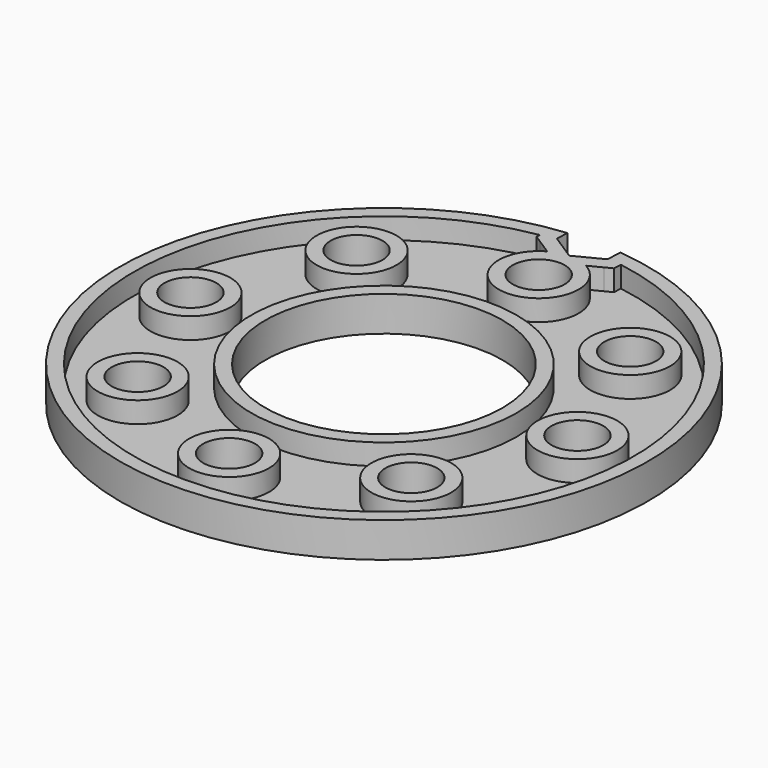
from build123d import *

# Parameters (mm, degrees)
F0_R        = 4.7064707614
F0_R_2      = 21.5186597363
F1_DEPTH    = 6.35
F2_T        = 2.54
F2_T3_DEPTH = 11.43


# Not quite as in the source:
# - a shell that OpenCascade refuses in one call is made with other operations: the cavity is built on its own and cut out


with BuildPart() as f1:
    # F0 (on Top) → F1 (new body)
    with BuildSketch(Plane.XY):
        with BuildLine():
            Line((-4.9161130278, 45.3357483006), (-4.8021092029, 47.6136840266))
            ThreePointArc((-4.8021092029, 47.6136840266), (0.0120888652, -47.8552297376), (4.7780528964, 47.6161041025))
            Line((4.7780528964, 47.6161041025), (4.639992765, 44.8574939765))
            Line((4.639992765, 44.8574939765), (-0.2761202627, 42.3380110126))
            Line((-0.2761202627, 42.3380110126), (-4.9161130278, 45.3357483006))
        make_face()
        with Locations((-24.80855963, -24.80855963)):
            Circle(F0_R, mode=Mode.SUBTRACT)
        with Locations((0, -35.0846014917)):
            Circle(F0_R, mode=Mode.SUBTRACT)
        with Locations((24.80855963, -24.80855963)):
            Circle(F0_R, mode=Mode.SUBTRACT)
        with Locations((-35.0846014917, 0)):
            Circle(F0_R, mode=Mode.SUBTRACT)
        with Locations((-24.80855963, 24.80855963)):
            Circle(F0_R, mode=Mode.SUBTRACT)
        Circle(F0_R_2, mode=Mode.SUBTRACT)
        with Locations((35.0846014917, 0)):
            Circle(F0_R, mode=Mode.SUBTRACT)
        with Locations((0, 35.0846014917)):
            Circle(F0_R, mode=Mode.SUBTRACT)
        with Locations((24.80855963, 24.80855963)):
            Circle(F0_R, mode=Mode.SUBTRACT)
    extrude(amount=F1_DEPTH)

    # F2: shell of thickness 2.54, made by hand


with BuildPart() as f2_core1:
    # F2_t2: copy of F1
    add(f1.part)

    # the walls: a layer under each face that stays
    f2_faces = [f2_core1.faces().sort_by_distance(p)[0] for p in [
        (-2.5961166453, 43.8368796566, 3.175),
        (-4.8591111154, 46.4747161636, 3.175),
        (0.0120888652, -47.8552297376, 3.175),
        (4.7090228307, 46.2367990395, 3.175),
        (2.1819362512, 43.5977524946, 3.175),
        (-29.5150303914, -24.80855963, 3.175),
        (-4.7064707614, -35.0846014917, 3.175),
        (20.1020888686, -24.80855963, 3.175),
        (-39.7910722531, 0, 3.175),
        (-29.5150303914, 24.80855963, 3.175),
        (-21.5186597363, 0, 3.175),
        (30.3781307302, 0, 3.175),
        (-4.7064707614, 35.0846014917, 3.175),
        (20.1020888686, 24.80855963, 3.175),
        (-31.9034875097, -31.9433420367, 0),
    ]]
    thicken(f2_faces, amount=-F2_T, mode=Mode.SUBTRACT)

    # F2_s4 → F2_t3 (cut)
    with BuildSketch(Plane.XY.offset(-2.54)):
        Polygon((-0.2739212432, 42.3819501104), (-1.6544837368, 40.2045363506), (-0.4227215664, 39.4087378278), (0.8823412559, 40.0775758974), align=None)
        Polygon((-4.8769611431, 45.3558134427), (-6.2944765018, 43.2022736386), (-7.5262386722, 43.9980721614), (-7.4529380204, 45.4627087538), align=None)
        Polygon((4.6030398999, 44.8813679322), (7.1768177577, 44.7305335234), (7.1035171059, 43.265896931), (5.7984542836, 42.5970588614), align=None)
    extrude(amount=F2_T3_DEPTH, mode=Mode.SUBTRACT)


with BuildPart() as f1_1:
    add(f1.part)

    # what is left inside the walls is the cavity
    f2_cavity = [f2_core1.part.solids().sort_by_distance(p)[0] for p in [
        (-22.657616, 14.723726, 2.5654),
    ]]
    add(f2_cavity, mode=Mode.SUBTRACT)


solid = f1_1.part
